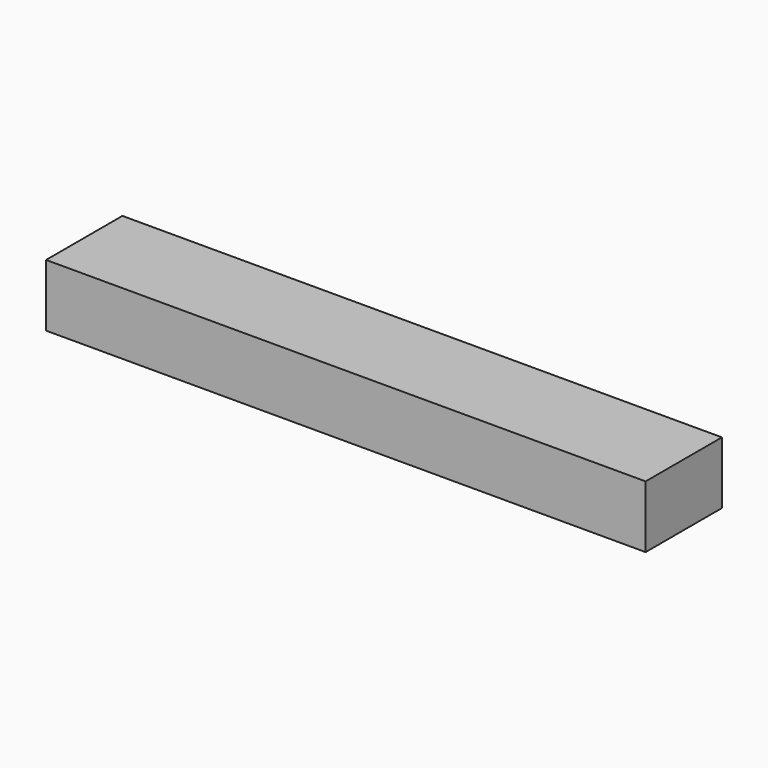
from build123d import *

# Parameters (mm, degrees)
F0_W     = 489.0587627888
F0_H     = 77.809035778
F1_DEPTH = 50.8


# Not quite as in the source:
# - a feature names something its author has since deleted; it is built from what else it names


with BuildPart() as f1:
    # F0 (on Top) → F1 (new body)
    with BuildSketch(Plane.XY):
        Rectangle(F0_W, F0_H)
    extrude(amount=F1_DEPTH)


solid = f1.part
